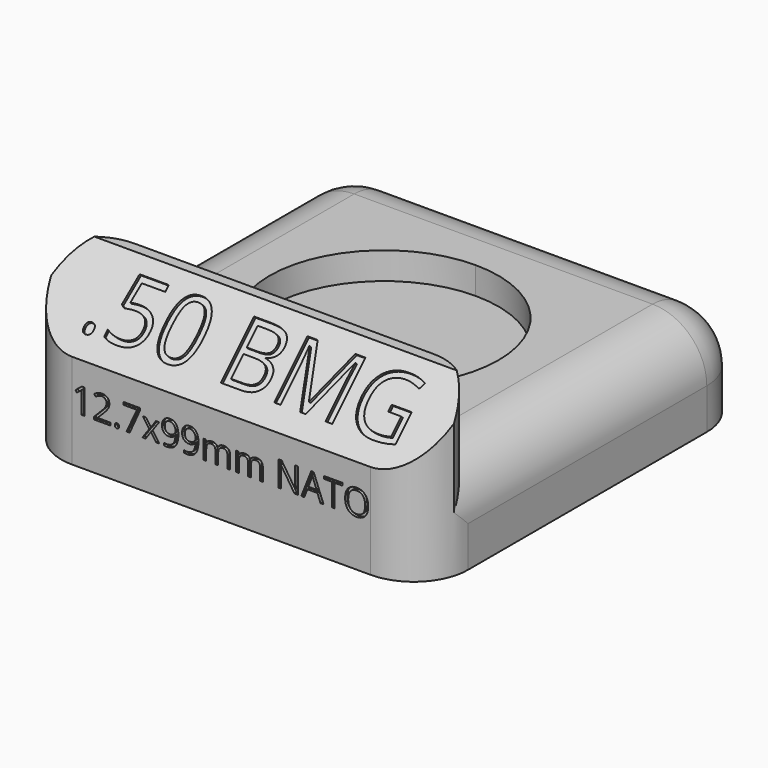
from build123d import *

# Parameters (mm, degrees)
F1_DEPTH      = 6.35
F2_DEPTH      = 8.89
F3_W          = 38.1
F3_H          = 7.3315937917
F4_DEPTH      = 6.35
F5_SIZE       = 6.35
F6_T1_DEPTH   = 34.29
F6_T3_DEPTH   = 25.6884062083
F6_T5_DEPTH   = 27.94
F6_T7_DEPTH   = 19.05
F6_T9_DEPTH   = 16.51
F6_S13_W      = 5.08
F6_S13_H      = 5.08
F6_T14_DEPTH  = 5.08
F6_S19_W      = 5.08
F6_S19_H      = 5.08
F6_T20_DEPTH  = 5.08
F6_T27_DEPTH  = 31.75
F6_T31_DEPTH  = 38.3884062083
F6_T38_DEPTH  = 31.75
F6_T42_DEPTH  = 38.3884062083
F7_TEXT_SIZE  = 7.701282286
F8_DEPTH      = 0.254
F9_TEXT_SIZE  = 3.2903855
F10_DEPTH     = 0.254
F11_TEXT_SIZE = 3.7188253889
F12_DEPTH     = 0.254


# Not quite as in the source:
# - a fillet or chamfer that OpenCascade refuses, or shapes differently, is made with other operations: its cross-section is extruded or revolved along the edge and cut away or added
# - Text() gives the source's letters only with a copy of the font that has no kerning and outlines rounded to 1/6400 em; it was checked with that copy


with BuildPart() as f1:
    # F0 (on Top) → F1 (new body)
    with BuildSketch(Plane.XY):
        with BuildLine():
            Line((-33.0781055778, -30.627979084), (-33.0781055778, -30.119979084))
            ThreePointArc((-33.0781055778, -30.119979084), (-43.7969055778, -40.838779084), (-33.0781055778, -51.557579084))
            Line((-33.0781055778, -51.557579084), (-33.0781055778, -51.049579084))
            ThreePointArc((-33.0781055778, -51.049579084), (-43.2889055778, -40.838779084), (-33.0781055778, -30.627979084))
        make_face()
        Polygon((-39.4281055778, -59.888779084), (-52.1281055778, -47.188779084), (-52.1281055778, -59.888779084), align=None)
        with BuildLine():
            Line((-33.0781055778, -51.049579084), (-33.0781055778, -30.627979084))
            ThreePointArc((-33.0781055778, -30.627979084), (-43.2889055778, -40.838779084), (-33.0781055778, -51.049579084))
        make_face()
        with BuildLine():
            ThreePointArc((-22.8673055778, -40.838779084), (-25.8579796565, -33.6186531626), (-33.0781055778, -30.627979084))
            Line((-33.0781055778, -30.627979084), (-33.0781055778, -51.049579084))
            ThreePointArc((-33.0781055778, -51.049579084), (-25.8579796565, -48.0589050053), (-22.8673055778, -40.838779084))
        make_face()
        Polygon((-14.0281055778, -21.788779084), (-26.7281055778, -21.788779084), (-14.0281055778, -34.488779084), align=None)
        Polygon((-14.0281055778, -59.888779084), (-14.0281055778, -47.188779084), (-26.7281055778, -59.888779084), align=None)
        with BuildLine():
            Line((-33.0781055778, -21.788779084), (-39.4281055778, -21.788779084))
            Line((-39.4281055778, -21.788779084), (-52.1281055778, -34.488779084))
            Line((-52.1281055778, -34.488779084), (-52.1281055778, -47.188779084))
            Line((-52.1281055778, -47.188779084), (-39.4281055778, -59.888779084))
            Line((-39.4281055778, -59.888779084), (-33.0781055778, -59.888779084))
            Line((-33.0781055778, -59.888779084), (-33.0781055778, -51.557579084))
            ThreePointArc((-33.0781055778, -51.557579084), (-43.7969055778, -40.838779084), (-33.0781055778, -30.119979084))
            Line((-33.0781055778, -30.119979084), (-33.0781055778, -21.788779084))
        make_face()
        with BuildLine():
            Line((-26.7281055778, -21.788779084), (-33.0781055778, -21.788779084))
            Line((-33.0781055778, -21.788779084), (-33.0781055778, -30.119979084))
            ThreePointArc((-33.0781055778, -30.119979084), (-25.4987694116, -33.2594429178), (-22.3593055778, -40.838779084))
            ThreePointArc((-22.3593055778, -40.838779084), (-25.4987694116, -48.4181152501), (-33.0781055778, -51.557579084))
            Line((-33.0781055778, -51.557579084), (-33.0781055778, -59.888779084))
            Line((-33.0781055778, -59.888779084), (-26.7281055778, -59.888779084))
            Line((-26.7281055778, -59.888779084), (-14.0281055778, -47.188779084))
            Line((-14.0281055778, -47.188779084), (-14.0281055778, -34.488779084))
            Line((-14.0281055778, -34.488779084), (-26.7281055778, -21.788779084))
        make_face()
        Polygon((-39.4281055778, -21.788779084), (-52.1281055778, -21.788779084), (-52.1281055778, -34.488779084), align=None)
        with BuildLine():
            ThreePointArc((-22.3593055778, -40.838779084), (-25.4987694116, -33.2594429178), (-33.0781055778, -30.119979084))
            Line((-33.0781055778, -30.119979084), (-33.0781055778, -30.627979084))
            ThreePointArc((-33.0781055778, -30.627979084), (-25.8579796565, -33.6186531626), (-22.8673055778, -40.838779084))
            ThreePointArc((-22.8673055778, -40.838779084), (-25.8579796565, -48.0589050053), (-33.0781055778, -51.049579084))
            Line((-33.0781055778, -51.049579084), (-33.0781055778, -51.557579084))
            ThreePointArc((-33.0781055778, -51.557579084), (-25.4987694116, -48.4181152501), (-22.3593055778, -40.838779084))
        make_face()
    extrude(amount=F1_DEPTH)

    # F0 (on Top) → F2 (join)
    with BuildSketch(Plane.XY):
        with BuildLine():
            Line((-33.0781055778, -21.788779084), (-39.4281055778, -21.788779084))
            Line((-39.4281055778, -21.788779084), (-52.1281055778, -34.488779084))
            Line((-52.1281055778, -34.488779084), (-52.1281055778, -47.188779084))
            Line((-52.1281055778, -47.188779084), (-39.4281055778, -59.888779084))
            Line((-39.4281055778, -59.888779084), (-33.0781055778, -59.888779084))
            Line((-33.0781055778, -59.888779084), (-33.0781055778, -51.557579084))
            ThreePointArc((-33.0781055778, -51.557579084), (-43.7969055778, -40.838779084), (-33.0781055778, -30.119979084))
            Line((-33.0781055778, -30.119979084), (-33.0781055778, -21.788779084))
        make_face()
        with BuildLine():
            Line((-26.7281055778, -21.788779084), (-33.0781055778, -21.788779084))
            Line((-33.0781055778, -21.788779084), (-33.0781055778, -30.119979084))
            ThreePointArc((-33.0781055778, -30.119979084), (-25.4987694116, -33.2594429178), (-22.3593055778, -40.838779084))
            ThreePointArc((-22.3593055778, -40.838779084), (-25.4987694116, -48.4181152501), (-33.0781055778, -51.557579084))
            Line((-33.0781055778, -51.557579084), (-33.0781055778, -59.888779084))
            Line((-33.0781055778, -59.888779084), (-26.7281055778, -59.888779084))
            Line((-26.7281055778, -59.888779084), (-14.0281055778, -47.188779084))
            Line((-14.0281055778, -47.188779084), (-14.0281055778, -34.488779084))
            Line((-14.0281055778, -34.488779084), (-26.7281055778, -21.788779084))
        make_face()
        Polygon((-39.4281055778, -59.888779084), (-52.1281055778, -47.188779084), (-52.1281055778, -59.888779084), align=None)
        Polygon((-14.0281055778, -59.888779084), (-14.0281055778, -47.188779084), (-26.7281055778, -59.888779084), align=None)
        Polygon((-14.0281055778, -21.788779084), (-26.7281055778, -21.788779084), (-14.0281055778, -34.488779084), align=None)
        Polygon((-39.4281055778, -21.788779084), (-52.1281055778, -21.788779084), (-52.1281055778, -34.488779084), align=None)
    extrude(amount=F2_DEPTH)

    # F3 (on face) → F4 (join)
    with BuildSketch(Plane.XY.offset(8.89)):
        with Locations((-33.0781055778, -56.2229821881)):
            Rectangle(F3_W, F3_H)
    extrude(amount=F4_DEPTH)

    # F5
    f5_edges = [f1.edges().sort_by_distance(p)[0] for p in [
        (-33.078106, -59.888779, 15.24),
    ]]
    chamfer(f5_edges, length=F5_SIZE)

    # F6: fillet of radius 5.08 on 9 edges, made by hand

    # F6_s2 → F6_t1 (cut)
    with BuildSketch(Plane.XY.offset(-12.7)):
        with BuildLine():
            ThreePointArc((-47.0481055778, -59.888779084), (-50.6402080263, -58.4008815324), (-52.1281055778, -54.808779084))
            Line((-52.1281055778, -54.808779084), (-52.1281055778, -59.888779084))
            Line((-52.1281055778, -59.888779084), (-47.0481055778, -59.888779084))
        make_face()
        with BuildLine():
            ThreePointArc((-19.1081055778, -59.888779084), (-15.5160031294, -58.4008815324), (-14.0281055778, -54.808779084))
            Line((-14.0281055778, -54.808779084), (-14.0281055778, -59.888779084))
            Line((-14.0281055778, -59.888779084), (-19.1081055778, -59.888779084))
        make_face()
    extrude(amount=F6_T1_DEPTH, mode=Mode.SUBTRACT)

    # F6_s4 → F6_t3 (cut)
    with BuildSketch(Plane.XZ.offset(26.868779084)):
        with BuildLine():
            ThreePointArc((-14.0281055778, 3.81), (-15.5160031294, 7.4021024484), (-19.1081055778, 8.89))
            Line((-19.1081055778, 8.89), (-14.0281055778, 8.89))
            Line((-14.0281055778, 8.89), (-14.0281055778, 3.81))
        make_face()
        with BuildLine():
            ThreePointArc((-52.1281055778, 3.81), (-50.6402080263, 7.4021024484), (-47.0481055778, 8.89))
            Line((-47.0481055778, 8.89), (-52.1281055778, 8.89))
            Line((-52.1281055778, 8.89), (-52.1281055778, 3.81))
        make_face()
    extrude(amount=F6_T3_DEPTH, mode=Mode.SUBTRACT)

    # F6_s6 → F6_t5 (cut)
    with BuildSketch(Plane.YZ.offset(-47.0481055778)):
        with BuildLine():
            ThreePointArc((-26.868779084, 8.89), (-23.2766766355, 7.4021024484), (-21.788779084, 3.81))
            Line((-21.788779084, 3.81), (-21.788779084, 8.89))
            Line((-21.788779084, 8.89), (-26.868779084, 8.89))
        make_face()
    extrude(amount=F6_T5_DEPTH, mode=Mode.SUBTRACT)

    # F6_s8 → F6_t7 (cut)
    with BuildSketch(Plane.XY.offset(8.89)):
        with BuildLine():
            ThreePointArc((-52.1281055778, -57.6371852922), (-50.6402080263, -54.0450828438), (-47.0481055778, -52.5571852922))
            Line((-47.0481055778, -52.5571852922), (-52.1281055778, -52.5571852922))
            Line((-52.1281055778, -52.5571852922), (-52.1281055778, -57.6371852922))
        make_face()
        with BuildLine():
            ThreePointArc((-14.0281055778, -57.6371852922), (-15.5160031294, -54.0450828438), (-19.1081055778, -52.5571852922))
            Line((-19.1081055778, -52.5571852922), (-14.0281055778, -52.5571852922))
            Line((-14.0281055778, -52.5571852922), (-14.0281055778, -57.6371852922))
        make_face()
    extrude(amount=F6_T7_DEPTH, mode=Mode.SUBTRACT)

    # F6_s10 → F6_t9 (cut)
    with BuildSketch(Plane.XY.offset(-12.7)):
        with BuildLine():
            ThreePointArc((-52.1281055778, -26.868779084), (-50.6402080263, -23.2766766355), (-47.0481055778, -21.788779084))
            Line((-47.0481055778, -21.788779084), (-52.1281055778, -21.788779084))
            Line((-52.1281055778, -21.788779084), (-52.1281055778, -26.868779084))
        make_face()
        with BuildLine():
            ThreePointArc((-14.0281055778, -26.868779084), (-15.5160031294, -23.2766766355), (-19.1081055778, -21.788779084))
            Line((-19.1081055778, -21.788779084), (-14.0281055778, -21.788779084))
            Line((-14.0281055778, -21.788779084), (-14.0281055778, -26.868779084))
        make_face()
    extrude(amount=F6_T9_DEPTH, mode=Mode.SUBTRACT)


with BuildPart() as f6_tool12:
    # F6_s13 → F6_t14 (new body)
    with BuildSketch(Plane.XZ.offset(26.868779084)):
        with Locations((-16.5681055778, 6.35)):
            Rectangle(F6_S13_W, F6_S13_H)
    extrude(amount=-F6_T14_DEPTH)

    # F6_s15 → F6_t16 (revolve, cut)
    with BuildSketch(Plane(origin=(-19.1081055778, -26.868779084, 3.81), x_dir=(-0.7071067812, 0, -0.7071067812), z_dir=(0.7071067812, 0, -0.7071067812))):
        with BuildLine():
            ThreePointArc((0, -5.08), (5.08, 0), (0, 5.08))
            Line((0, 5.08), (0, -5.08))
        make_face()
    revolve(axis=Axis((-19.1081055778, -26.868779084, 3.81), (0, 1, 0)), mode=Mode.SUBTRACT)


with BuildPart() as f1_1:
    add(f1.part)

    # F6_t11: cut F6_tool12
    add(f6_tool12.part, mode=Mode.SUBTRACT)


with BuildPart() as f6_tool18:
    # F6_s19 → F6_t20 (new body)
    with BuildSketch(Plane.XZ.offset(26.868779084)):
        with Locations((-49.5881055778, 6.35)):
            Rectangle(F6_S19_W, F6_S19_H)
    extrude(amount=-F6_T20_DEPTH)

    # F6_s21 → F6_t22 (revolve, cut)
    with BuildSketch(Plane(origin=(-47.0481055778, -26.868779084, 3.81), x_dir=(0.7071067812, 0, -0.7071067812), z_dir=(0.7071067812, 0, 0.7071067812))):
        with BuildLine():
            ThreePointArc((0, -5.08), (5.08, 0), (0, 5.08))
            Line((0, 5.08), (0, -5.08))
        make_face()
    revolve(axis=Axis((-47.0481055778, -26.868779084, 3.81), (0, 1, 0)), mode=Mode.SUBTRACT)


with BuildPart() as f1_2:
    add(f1_1.part)

    # F6_t17: cut F6_tool18
    add(f6_tool18.part, mode=Mode.SUBTRACT)


with BuildPart() as f6_tool25:
    # F6_s26 → F6_t27 (new body)
    with BuildSketch(Plane.XY.offset(-3.81)):
        with BuildLine():
            ThreePointArc((-14.0281055778, -57.6371852922), (-15.5160031294, -54.0450828438), (-19.1081055778, -52.5571852922))
            Line((-19.1081055778, -52.5571852922), (-14.0281055778, -52.5571852922))
            Line((-14.0281055778, -52.5571852922), (-14.0281055778, -57.6371852922))
        make_face()
    extrude(amount=F6_T27_DEPTH)

    split(bisect_by=Plane.XY.offset(8.89), keep=Keep.BOTTOM)


with BuildPart() as f6_tool29:
    # F6_s30 → F6_t31 (new body)
    with BuildSketch(Plane.XZ.offset(65.2571852922)):
        with BuildLine():
            ThreePointArc((-14.0281055778, 3.81), (-15.5160031294, 7.4021024484), (-19.1081055778, 8.89))
            Line((-19.1081055778, 8.89), (-14.0281055778, 8.89))
            Line((-14.0281055778, 8.89), (-14.0281055778, 3.81))
        make_face()
    extrude(amount=-F6_T31_DEPTH)

    split(bisect_by=Plane.XZ.offset(52.5571852922), keep=Keep.TOP)


with BuildPart() as f6_tool25_1:
    add(f6_tool25.part)

    # F6_t33: intersect F6_tool29
    add(f6_tool29.part, mode=Mode.INTERSECT)


with BuildPart() as f1_3:
    add(f1_2.part)

    # F6_t23: cut F6_tool25
    add(f6_tool25_1.part, mode=Mode.SUBTRACT)


with BuildPart() as f6_tool36:
    # F6_s37 → F6_t38 (new body)
    with BuildSketch(Plane.XY.offset(-3.81)):
        with BuildLine():
            ThreePointArc((-52.1281055778, -57.6371852922), (-50.6402080263, -54.0450828438), (-47.0481055778, -52.5571852922))
            Line((-47.0481055778, -52.5571852922), (-52.1281055778, -52.5571852922))
            Line((-52.1281055778, -52.5571852922), (-52.1281055778, -57.6371852922))
        make_face()
    extrude(amount=F6_T38_DEPTH)

    split(bisect_by=Plane.XY.offset(8.89), keep=Keep.BOTTOM)


with BuildPart() as f6_tool40:
    # F6_s41 → F6_t42 (new body)
    with BuildSketch(Plane.XZ.offset(26.868779084)):
        with BuildLine():
            ThreePointArc((-52.1281055778, 3.81), (-50.6402080263, 7.4021024484), (-47.0481055778, 8.89))
            Line((-47.0481055778, 8.89), (-52.1281055778, 8.89))
            Line((-52.1281055778, 8.89), (-52.1281055778, 3.81))
        make_face()
    extrude(amount=F6_T42_DEPTH)

    split(bisect_by=Plane.XZ.offset(52.5571852922), keep=Keep.TOP)


with BuildPart() as f6_tool36_1:
    add(f6_tool36.part)

    # F6_t44: intersect F6_tool40
    add(f6_tool40.part, mode=Mode.INTERSECT)


with BuildPart() as f1_4:
    add(f1_3.part)

    # F6_t34: cut F6_tool36
    add(f6_tool36_1.part, mode=Mode.SUBTRACT)

    # F7 (on face) → F8 (cut)
    with BuildSketch(Plane(origin=(0, -34.389389542, 34.389389542), x_dir=(1, 0, 0), z_dir=(0, -0.7071067812, 0.7071067812))):
        with Locations((-47.8718057275, -34.0406820178)):
            Text('.50 BMG', F7_TEXT_SIZE, font='Open Sans', text_align=(TextAlign.LEFT, TextAlign.BOTTOM))
    extrude(amount=-F8_DEPTH, mode=Mode.SUBTRACT)

    # F9 (on face) → F10 (cut)
    with BuildSketch(Plane.XZ.offset(59.888779084)):
        with Locations((-47.0481055778, 4.3830258351)):
            Text('12.7x99mm NATO', F9_TEXT_SIZE, font='Open Sans', text_align=(TextAlign.LEFT, TextAlign.BOTTOM))
    extrude(amount=-F10_DEPTH, mode=Mode.SUBTRACT)

    # F11 (on face) → F12 (cut)
    with BuildSketch(Plane(origin=(0, 0, 0), x_dir=(1, 0, 0), z_dir=(0, 0, -1))):
        with Locations((-47.0481055778, 52.131224804)):
            Text('Cristian Quinata', F11_TEXT_SIZE, font='Open Sans', text_align=(TextAlign.LEFT, TextAlign.BOTTOM))
    extrude(amount=-F12_DEPTH, mode=Mode.SUBTRACT)


solid = f1_4.part
